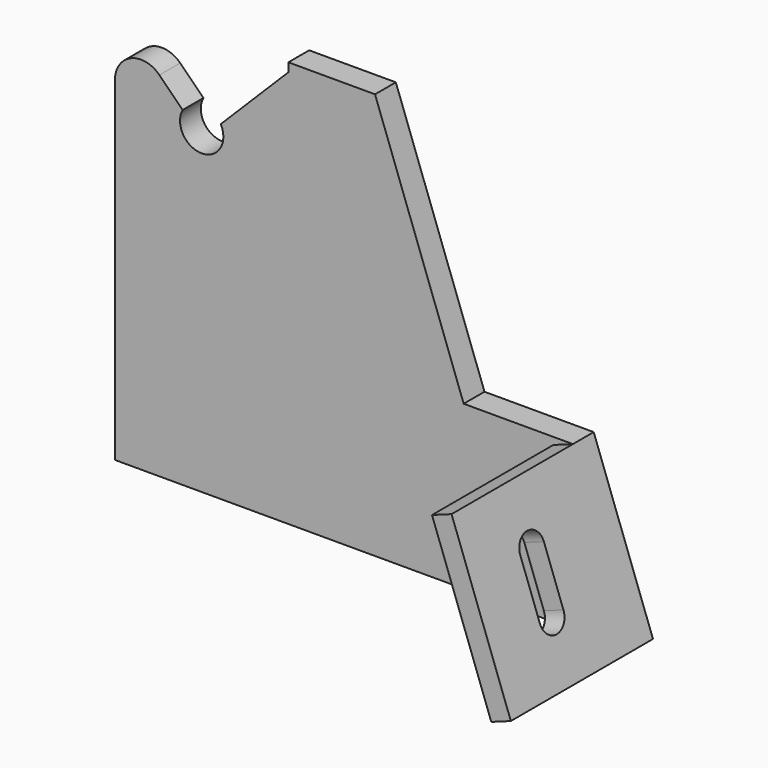
from build123d import *

# Parameters (mm, degrees)
F1_DEPTH = 22.225
F2_W     = 4.318
F2_H     = 12.7
F3_DEPTH = 11.212402643
F4_R     = 2.15899
F5_R     = 3.175
F6_DEPTH = 3.81
F8_DEPTH = 25.4
F9_R     = 3.81


# Not quite as in the source:
# - a fillet or chamfer is up to 0.001 mm smaller than in the source, because OpenCascade refuses the exact size


with BuildPart() as f1:
    # F0 (on Front) → F1 (new body)
    with BuildSketch(Plane.XZ):
        Polygon((11.5514947486, -84.959096284), (2.8641831082, -61.090903716), (0, -62.1333811129), (8.6873116405, -86.0015736808), align=None)
    extrude(amount=F1_DEPTH)

    # F2 (on face) → F3 (cut, through all)
    with BuildSketch(Plane(origin=(-19.9692837636, 0, -7.2682248896), x_dir=(0, -1, 0), z_dir=(-0.9396926208, 0, -0.3420201433))):
        with Locations((11.1125, -71.0862797362)):
            Rectangle(F2_W, F2_H)
        with Locations((11.1125, -93.3112797362)):
            Rectangle(F2_W, F2_H)
    extrude(amount=-F3_DEPTH, mode=Mode.SUBTRACT)

    # F4 (radius 2.159 in the source; OpenCascade refuses exactly that, so slightly less here)
    f4_edges = [f1.edges().sort_by_distance(p)[0] for p in [
        (3.603919, -8.9535, -67.579191),
        (3.603919, -13.2715, -67.579191),
        (7.947575, -13.2715, -79.513287),
        (7.947575, -8.9535, -79.513287),
    ]]
    fillet(f4_edges, radius=F4_R)

    # F5 (on Front) → F6 (join)
    with BuildSketch(Plane.XZ):
        Polygon((11.5514947486, -84.959096284), (2.8641831082, -61.090903716), (-13.1392344849, -61.090903716), (-26.1296610716, -25.4), (-64.2296610716, -25.4), (-64.2296610716, -84.959096284), align=None)
        with Locations((-51.5296610716, -38.1)):
            Circle(F5_R, mode=Mode.SUBTRACT)
    extrude(amount=-F6_DEPTH)

    # F7 (on Front) → F8 (cut)
    with BuildSketch(Plane.XZ):
        Polygon((-65.5156196266, -25.4), (-51.5296610716, -39.3859585549), (-38.8296610716, -26.6859585549), (-38.8296610716, -25.4), align=None)
    extrude(amount=-F8_DEPTH, mode=Mode.SUBTRACT)

    # F9
    f9_edges = [f1.edges().sort_by_distance(p)[0] for p in [
        (-64.229661, 1.905, -26.685959),
    ]]
    fillet(f9_edges, radius=F9_R)


solid = f1.part
